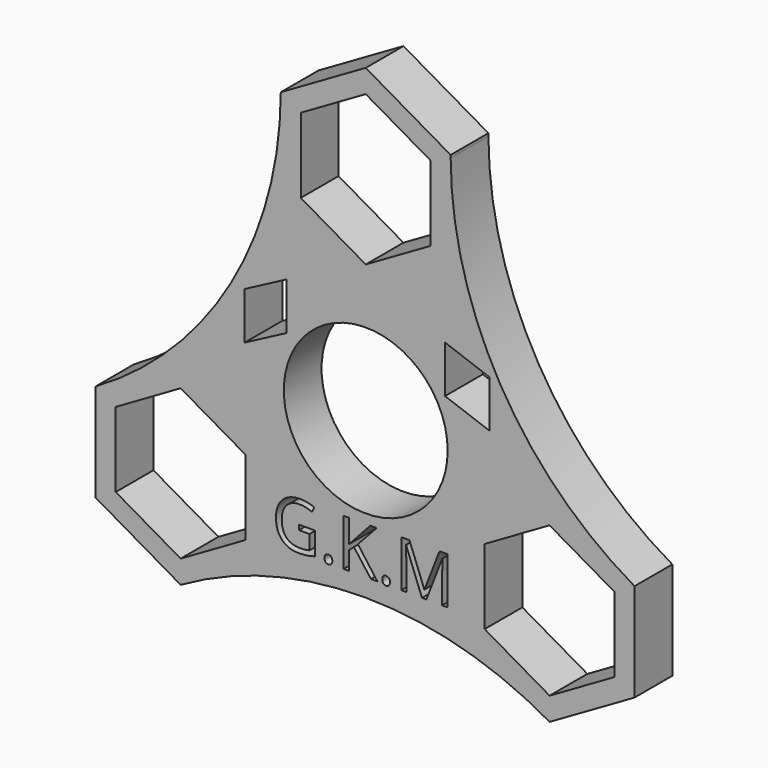
from build123d import *

# Parameters (mm, degrees)
F0_R         = 14.2875
F0_R_2       = 11.0236
F1_DEPTH     = 6.35
F2_TEXT_SIZE = 8.8194444444
F3_DEPTH     = 25.4
F5_DEPTH     = 25.4


# Not quite as in the source:
# - Text() gives the source's letters only with a copy of the font that has no kerning and outlines rounded to 1/6400 em; it was checked with that copy


with BuildPart() as f1:
    # F0 (on Front) → F1 (new body)
    with BuildSketch(Plane.XZ):
        with BuildLine():
            Line((0, 15.3767728463), (-11.43, 21.9758864232))
            Line((-11.43, 21.9758864232), (-11.43, 35.1741135768))
            ThreePointArc((-11.43, 35.1741135768), (-18.1503993358, 10.3771608603), (-36.3343377884, -7.7721370217))
            Line((-36.3343377884, -7.7721370217), (-24.9043377884, -1.1730234449))
            Line((-24.9043377884, -1.1730234449), (-13.4743377884, -7.7721370217))
            Line((-13.4743377884, -7.7721370217), (-13.4743377884, -20.9703641754))
            Line((-13.4743377884, -20.9703641754), (-24.9043377884, -27.5694777523))
            ThreePointArc((-24.9043377884, -27.5694777523), (-0.0693471315, -20.9910379424), (24.7403751215, -27.6641416421))
            Line((24.7403751215, -27.6641416421), (13.3103751215, -21.0650280653))
            Line((13.3103751215, -21.0650280653), (13.3103751215, -7.8668009116))
            Line((13.3103751215, -7.8668009116), (24.7403751215, -1.2676873348))
            Line((24.7403751215, -1.2676873348), (36.1703751215, -7.8668009116))
            ThreePointArc((36.1703751215, -7.8668009116), (18.1061542486, 10.1630074539), (11.43, 34.7967044946))
            Line((11.43, 34.7967044946), (11.43, 21.9758864232))
            Line((11.43, 21.9758864232), (0, 15.3767728463))
        make_face()
        with Locations((-0.0063007916, -0.1784144884)):
            Circle(F0_R, mode=Mode.SUBTRACT)
        with Locations((-0.0063007916, -0.1784144884)):
            Circle(F0_R)
        Circle(F0_R_2, mode=Mode.SUBTRACT)
        Polygon((-24.9043377884, -1.1730234449), (-36.3343377884, -7.7721370217), (-36.3343377884, -20.9703641754), (-24.9043377884, -27.5694777523), (-13.4743377884, -20.9703641754), (-13.4743377884, -7.7721370217), align=None)
        Polygon((-16.1667377884, -19.4159063107), (-24.9043377884, -24.4605620227), (-33.6419377884, -19.4159063107), (-33.6419377884, -9.3265948865), (-24.9043377884, -4.2819391744), (-16.1667377884, -9.3265948865), align=None, mode=Mode.SUBTRACT)
        Polygon((36.1703751215, -21.0650280653), (36.1703751215, -7.8668009116), (24.7403751215, -1.2676873348), (13.3103751215, -7.8668009116), (13.3103751215, -21.0650280653), (24.7403751215, -27.6641416421), align=None)
        Polygon((24.7403751215, -4.3766030643), (33.4779751215, -9.4212587764), (33.4779751215, -19.5105702005), (24.7403751215, -24.5552259126), (16.0027751215, -19.5105702005), (16.0027751215, -9.4212587764), align=None, mode=Mode.SUBTRACT)
        with BuildLine():
            Line((-11.43, 35.1741135768), (-11.43, 21.9758864232))
            Line((-11.43, 21.9758864232), (0, 15.3767728463))
            Line((0, 15.3767728463), (11.43, 21.9758864232))
            Line((11.43, 21.9758864232), (11.43, 34.7967044946))
            ThreePointArc((11.43, 34.7967044946), (11.429640173, 34.9854090357), (11.43, 35.1741135768))
            Line((11.43, 35.1741135768), (0, 41.7732271537))
            Line((0, 41.7732271537), (-11.43, 35.1741135768))
        make_face()
        Polygon((0, 18.4856885759), (-8.7376, 23.5303442879), (-8.7376, 33.6196557121), (0, 38.6643114241), (8.7376, 33.6196557121), (8.7376, 23.5303442879), align=None, mode=Mode.SUBTRACT)
    extrude(amount=F1_DEPTH)

    # F2 (on Front) → F3 (cut)
    with BuildSketch(Plane.XZ):
        with Locations((-12.610601472, -18.5568776757)):
            Text('G.K.M', F2_TEXT_SIZE, font='Open Sans', text_align=(TextAlign.LEFT, TextAlign.BOTTOM))
    extrude(amount=F3_DEPTH, mode=Mode.SUBTRACT)

    # F4 (on Front) → F5 (cut)
    with BuildSketch(Plane.XZ):
        Polygon((-10.668, 6.8895352678), (-10.668, 13.2395352678), (-16.2879870804, 10.283482965), (-16.2879870804, 3.933482965), align=None)
        Polygon((16.6426125939, 10.5573119393), (10.668, 12.7082429826), (10.668, 6.3582429826), (16.6426125939, 4.2073119393), align=None)
    extrude(amount=F5_DEPTH, mode=Mode.SUBTRACT)


solid = f1.part
